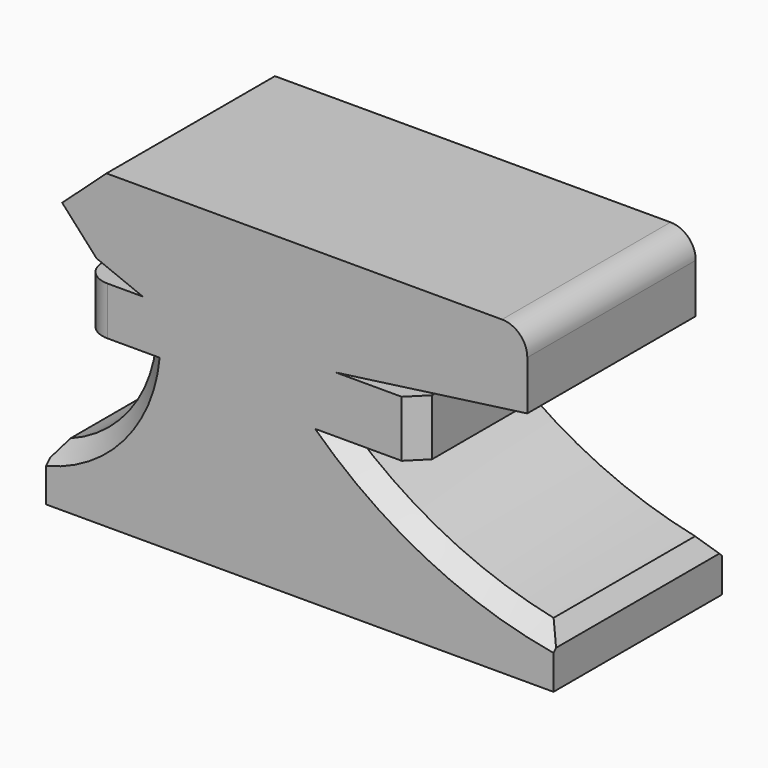
from build123d import *

# Parameters (mm, degrees)
F1_DEPTH     = 31.75
F2_T1_DEPTH  = 42.6160723951
F2_T3_DEPTH  = 41.3681408406
F2_T8_ANGLE  = 42.4045514756
F2_T13_ANGLE = 42.4045514756
F2_T18_ANGLE = 105.7775701063
F2_T23_ANGLE = 105.7775701063
F2_T28_DEPTH = 21.5661635602
F2_T33_DEPTH = 21.5661635602
F3_R         = 3.81


# Not quite as in the source:
# - a fillet or chamfer that OpenCascade refuses, or shapes differently, is made with other operations: its cross-section is extruded or revolved along the edge and cut away or added


with BuildPart() as f1:
    # F0 (on Front) → F1 (new body)
    with BuildSketch(Plane.XZ):
        with BuildLine():
            Line((-34.918975085, 0), (0, 0))
            Line((0, 0), (41.5991283953, 0))
            Line((41.5991283953, 0), (41.5991283953, 7.7429031953))
            ThreePointArc((41.5991283953, 7.7429031953), (24.4471014125, 13.2848832085), (9.4129433855, 23.2287086546))
            Line((9.4129433855, 23.2287086546), (21.2550275028, 23.2287086546))
            Line((21.2550275028, 23.2287086546), (21.2550275028, 31.730722636))
            Line((21.2550275028, 31.730722636), (8.8056568056, 31.730722636))
            Line((8.8056568056, 31.730722636), (37.6517660916, 35.6780849397))
            Line((37.6517660916, 35.6780849397), (37.6517660916, 46.912882477))
            Line((37.6517660916, 46.912882477), (-25.8096773177, 46.912882477))
            Line((-25.8096773177, 46.912882477), (-32.4898287654, 40.8400185406))
            Line((-32.4898287654, 40.8400185406), (-27.3100329334, 35.1422421722))
            Line((-27.3100329334, 35.1422421722), (-20.3440990299, 32.3380082846))
            Line((-20.3440990299, 32.3380082846), (-29.4533986598, 32.3380082846))
            Line((-29.4533986598, 32.3380082846), (-29.4533986598, 25.0505693257))
            Line((-29.4533986598, 25.0505693257), (-20.3440990299, 25.0505693257))
            ThreePointArc((-20.3440990299, 25.0505693257), (-24.9642185282, 14.1505733942), (-34.918975085, 7.7429031953))
            Line((-34.918975085, 7.7429031953), (-34.918975085, 0))
        make_face()
    extrude(amount=F1_DEPTH)

    # F2: chamfer of 2.54 on 8 edges, made by hand

    # F2_s2 → F2_t1 (cut)
    with BuildSketch(Plane.XZ.offset(-5.4330361975)):
        with BuildLine():
            Line((39.5823851634, 8.1350460371), (41.5991283953, 5.6495275088))
            Line((41.5991283953, 5.6495275088), (41.5991283953, 7.7429031953))
            ThreePointArc((41.5991283953, 7.7429031953), (40.55098868, 7.9386371476), (39.5823851634, 8.1350460371))
        make_face()
    extrude(amount=F2_T1_DEPTH, mode=Mode.SUBTRACT)

    # F2_s4 → F2_t3 (cut)
    with BuildSketch(Plane.XZ.offset(-4.8090704203)):
        with BuildLine():
            Line((-34.918975085, 5.9036651076), (-33.2718375789, 8.2815626174))
            ThreePointArc((-33.2718375789, 8.2815626174), (-34.0510462722, 8.0071201362), (-34.918975085, 7.7429031953))
            Line((-34.918975085, 7.7429031953), (-34.918975085, 5.9036651076))
        make_face()
    extrude(amount=F2_T3_DEPTH, mode=Mode.SUBTRACT)


with BuildPart() as f2_tool6:
    # F2_s7 → F2_t8 (revolve)
    with BuildSketch(Plane(origin=(47.2414051796, 0, -3.7108637316), x_dir=(0, 1, 0), z_dir=(0.9969290674, 0, -0.078309862))):
        Polygon((-31.75, 8.1162253666), (-29.21, 10.6562253666), (-31.75, 10.6562253666), align=None)
    revolve(axis=Axis((53.2845253443, -31.75, 73.221491886), (0, 1, 0)), revolution_arc=F2_T8_ANGLE)

    split(bisect_by=Plane.XY.offset(23.2287086546), keep=Keep.BOTTOM)


with BuildPart() as f1_1:
    add(f1.part)

    # F2_t5: cut F2_tool6
    add(f2_tool6.part, mode=Mode.SUBTRACT)


with BuildPart() as f2_tool11:
    # F2_s12 → F2_t13 (revolve)
    with BuildSketch(Plane(origin=(47.2414051796, 0, -3.7108637316), x_dir=(0, 1, 0), z_dir=(0.9969290674, 0, -0.078309862))):
        Polygon((-2.54, 10.6562253666), (0, 8.1162253666), (0, 10.6562253666), align=None)
    revolve(axis=Axis((53.2845253443, 0, 73.221491886), (0, 1, 0)), revolution_arc=F2_T13_ANGLE)

    split(bisect_by=Plane.XY.offset(23.2287086546), keep=Keep.BOTTOM)


with BuildPart() as f1_2:
    add(f1_1.part)

    # F2_t10: cut F2_tool11
    add(f2_tool11.part, mode=Mode.SUBTRACT)


with BuildPart() as f2_tool16:
    # F2_s17 → F2_t18 (revolve)
    with BuildSketch(Plane(origin=(-7.8247411196, 0, 34.4744832645), x_dir=(0, 1, 0), z_dir=(-0.2213421957, 0, 0.975196202))):
        Polygon((-31.75, 10.7019792675), (-29.21, 13.2419792675), (-31.75, 13.2419792675), align=None)
    revolve(axis=Axis((-40.3361011805, -31.75, 27.0953160709), (0, 1, 0)), revolution_arc=F2_T18_ANGLE)

    split(bisect_by=Plane.XY.offset(25.0505693257), keep=Keep.BOTTOM)


with BuildPart() as f1_3:
    add(f1_2.part)

    # F2_t15: cut F2_tool16
    add(f2_tool16.part, mode=Mode.SUBTRACT)


with BuildPart() as f2_tool21:
    # F2_s22 → F2_t23 (revolve)
    with BuildSketch(Plane(origin=(-7.8247411196, 0, 34.4744832645), x_dir=(0, 1, 0), z_dir=(-0.2213421957, 0, 0.975196202))):
        Polygon((-2.54, 13.2419792675), (0, 10.7019792675), (0, 13.2419792675), align=None)
    revolve(axis=Axis((-40.3361011805, 0, 27.0953160709), (0, 1, 0)), revolution_arc=F2_T23_ANGLE)

    split(bisect_by=Plane.XY.offset(25.0505693257), keep=Keep.BOTTOM)


with BuildPart() as f1_4:
    add(f1_3.part)

    # F2_t20: cut F2_tool21
    add(f2_tool21.part, mode=Mode.SUBTRACT)


with BuildPart() as f2_tool26:
    # F2_s27 → F2_t28 (new body)
    with BuildSketch(Plane.XY.offset(16.6966338652)):
        Polygon((18.7150275028, 0), (21.2550275028, -2.54), (21.2550275028, 0), align=None)
    extrude(amount=F2_T28_DEPTH)

    split(bisect_by=Plane(origin=(-4.1004226977, 0, 29.9646275548), x_dir=(0, 1, 0), z_dir=(0.1355785861, 0, -0.9907665956)), keep=Keep.TOP)


with BuildPart() as f1_5:
    add(f1_4.part)

    # F2_t25: cut F2_tool26
    add(f2_tool26.part, mode=Mode.SUBTRACT)


with BuildPart() as f2_tool31:
    # F2_s32 → F2_t33 (new body)
    with BuildSketch(Plane.XY.offset(16.6966338652)):
        Polygon((18.7150275028, -31.75), (21.2550275028, -29.21), (21.2550275028, -31.75), align=None)
    extrude(amount=F2_T33_DEPTH)

    split(bisect_by=Plane(origin=(-4.1004226977, 0, 29.9646275548), x_dir=(0, 1, 0), z_dir=(0.1355785861, 0, -0.9907665956)), keep=Keep.TOP)


with BuildPart() as f1_6:
    add(f1_5.part)

    # F2_t30: cut F2_tool31
    add(f2_tool31.part, mode=Mode.SUBTRACT)

    # F3
    f3_edges = [f1_6.edges().sort_by_distance(p)[0] for p in [
        (-29.453399, -31.75, 28.694289),
        (-29.453399, 0, 28.694289),
        (37.651766, -15.875, 46.912882),
    ]]
    fillet(f3_edges, radius=F3_R)


solid = f1_6.part
